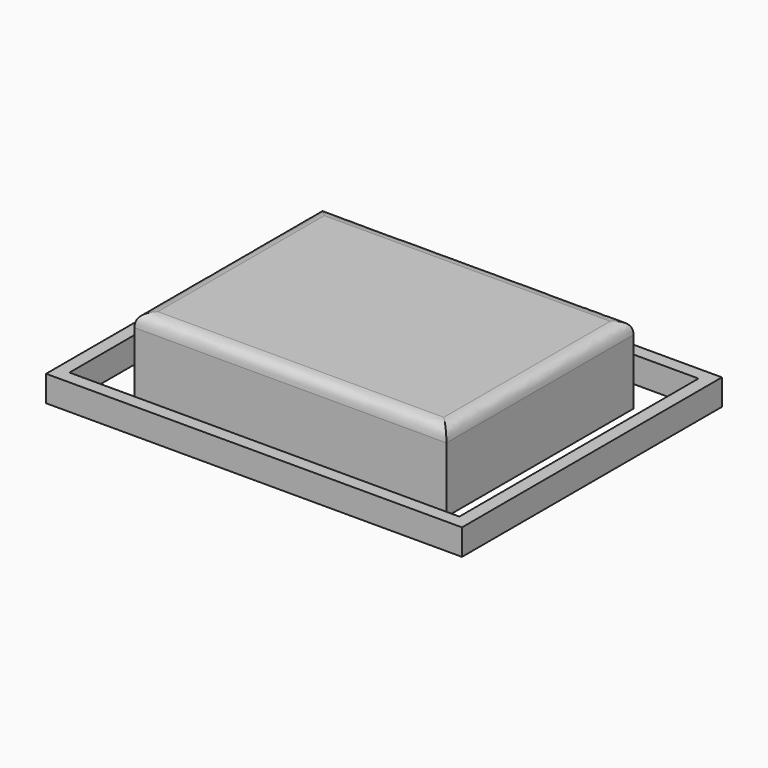
from build123d import *

# Parameters (mm, degrees)
F0_W        = 304.8
F0_H        = 228.6
F1_DEPTH    = 76.2
F2_T        = -6.35
F3_T1_DEPTH = 368.3
F3_T3_DEPTH = 292.1
F4_W        = 406.4
F4_H        = 317.5
F4_W_2      = 381
F4_H_2      = 292.1
F5_DEPTH    = 25.4


# Not quite as in the source:
# - a fillet or chamfer that OpenCascade refuses, or shapes differently, is made with other operations: its cross-section is extruded or revolved along the edge and cut away or added


with BuildPart() as f1:
    # F0 (on Top) → F1 (new body)
    with BuildSketch(Plane.XY):
        Rectangle(F0_W, F0_H)
    extrude(amount=F1_DEPTH)

    # F2
    f2_openings = [f1.faces().sort_by_distance(p)[0] for p in [
        (0, 0, 0),
    ]]
    offset(amount=F2_T, openings=f2_openings)

    # F3: fillet of radius 12.7 on 4 edges, made by hand

    # F3_s2 → F3_t1 (cut)
    with BuildSketch(Plane.YZ.offset(-184.15)):
        with BuildLine():
            add(Edge.make_bspline(
                [(-114.3, 63.5), (-114.3, 76.2), (-101.6, 76.2)],
                knots=[0, 0, 0, 1, 1, 1], degree=2, weights=[1, 1, 1]))
            Line((-101.6, 76.2), (-114.3, 76.2))
            Line((-114.3, 76.2), (-114.3, 63.5))
        make_face()
        with BuildLine():
            add(Edge.make_bspline(
                [(114.3, 63.5), (114.3, 76.2), (101.6, 76.2)],
                knots=[0, 0, 0, 1, 1, 1], degree=2, weights=[1, 1, 1]))
            Line((101.6, 76.2), (114.3, 76.2))
            Line((114.3, 76.2), (114.3, 63.5))
        make_face()
    extrude(amount=F3_T1_DEPTH, mode=Mode.SUBTRACT)

    # F3_s4 → F3_t3 (cut)
    with BuildSketch(Plane.XZ.offset(-146.05)):
        with BuildLine():
            add(Edge.make_bspline(
                [(152.4, 63.5), (152.4, 76.2), (139.7, 76.2)],
                knots=[0, 0, 0, 1, 1, 1], degree=2, weights=[1, 1, 1]))
            Line((139.7, 76.2), (152.4, 76.2))
            Line((152.4, 76.2), (152.4, 63.5))
        make_face()
        with BuildLine():
            add(Edge.make_bspline(
                [(-152.4, 63.5), (-152.4, 76.2), (-139.7, 76.2)],
                knots=[0, 0, 0, 1, 1, 1], degree=2, weights=[1, 1, 1]))
            Line((-139.7, 76.2), (-152.4, 76.2))
            Line((-152.4, 76.2), (-152.4, 63.5))
        make_face()
    extrude(amount=F3_T3_DEPTH, mode=Mode.SUBTRACT)


with BuildPart() as f5:
    # F4 (on Top) → F5 (new body)
    with BuildSketch(Plane.XY):
        Rectangle(F4_W, F4_H)
        Rectangle(F4_W_2, F4_H_2, mode=Mode.SUBTRACT)
    extrude(amount=F5_DEPTH)


solid = Compound([f1.part, f5.part])
